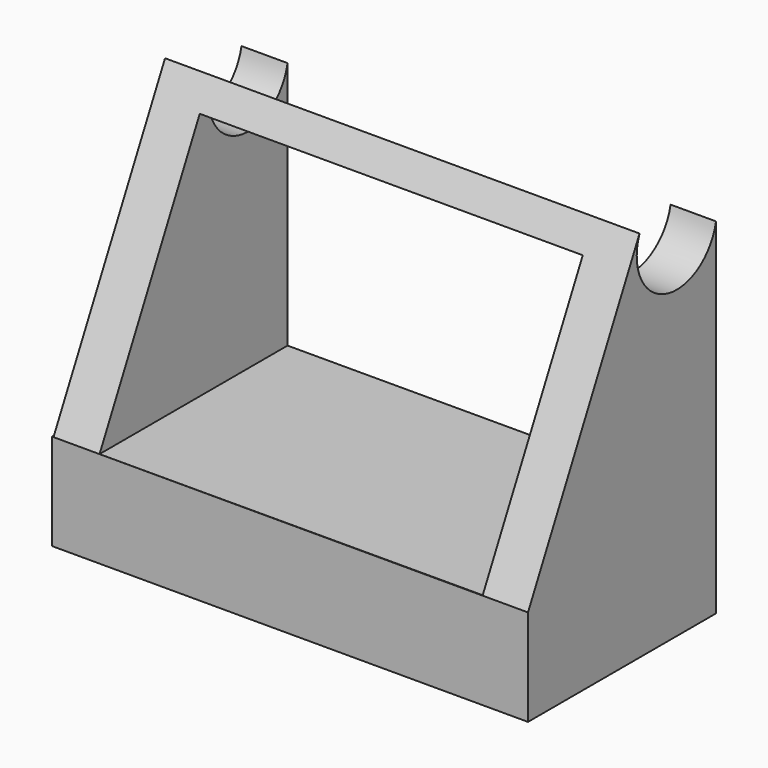
from build123d import *

# Parameters (mm, degrees)
F0_W      = 15.8
F0_H      = 7.8
F1_DEPTH  = 3.2
F3_DEPTH  = 1.5
F4_R      = 1.5020190756
F4_R_2    = 0.6083547137
F5_DEPTH  = 1.5
F7_DEPTH  = 15.75
F10_DEPTH = 25


# Not quite as in the source:
# - the program builds the solid bodies; features that only make, move or delete a surface that nothing else refers to are left out


with BuildPart() as f1:
    # F0 (on Top) → F1 (new body)
    with BuildSketch(Plane.XY):
        with Locations((-0.4272158258, 1.5226540988)):
            Rectangle(F0_W, F0_H)
    extrude(amount=F1_DEPTH)

    # F2 (on face) → F3 (cut)
    with BuildSketch(Plane(origin=(0, 0, 0), x_dir=(1, 0, 0), z_dir=(0, 0, -1))):
        Polygon((-0.8716915618, 0.8426669519), (-6.8171033636, 0.8426669519), (-6.8171033636, -1.5226540988), (-6.8171033636, -3.9279027842), (-0.4272158258, -3.9279027842), (5.9637515806, -3.9279027842), (5.9637515806, -1.5226540988), (5.9637515806, 0.8426669519), align=None)
    extrude(amount=-F3_DEPTH, mode=Mode.SUBTRACT)

    # F4 (on face) → F5 (join)
    with BuildSketch(Plane(origin=(0, 0, 1.5), x_dir=(1, 0, 0), z_dir=(0, 0, -1))):
        with Locations((-0.7097416674, -1.6585130943)):
            Circle(F4_R)
        with Locations((-0.7097416674, -1.6585130943)):
            Circle(F4_R_2, mode=Mode.SUBTRACT)
    extrude(amount=F5_DEPTH)

    # F6 (on face) → F7 (join)
    with BuildSketch(Plane.YZ.offset(7.4727841742)):
        with BuildLine():
            Line((-2.3773459012, 3.2), (5.4226540988, 3.2))
            Line((5.4226540988, 3.2), (5.4226540988, 11.4559076203))
            ThreePointArc((5.4226540988, 11.4559076203), (3.3247489231, 10.1865208896), (2.2503013028, 12.3906332074))
            Line((2.2503013028, 12.3906332074), (-2.3773459012, 3.2))
        make_face()
    extrude(amount=-F7_DEPTH)

    # F9 (on face) → F10 (cut)
    with BuildSketch(Plane(origin=(0, 5.4226540988, 0), x_dir=(-1, 0, 0), z_dir=(0, 1, 0))):
        Polygon((-5.9649683535, 11.4559076203), (-5.9649683535, 3.21011306), (6.7489589565, 3.2011167647), (6.7489589565, 11.4559076203), align=None)
    extrude(amount=-F10_DEPTH, mode=Mode.SUBTRACT)


solid = f1.part
